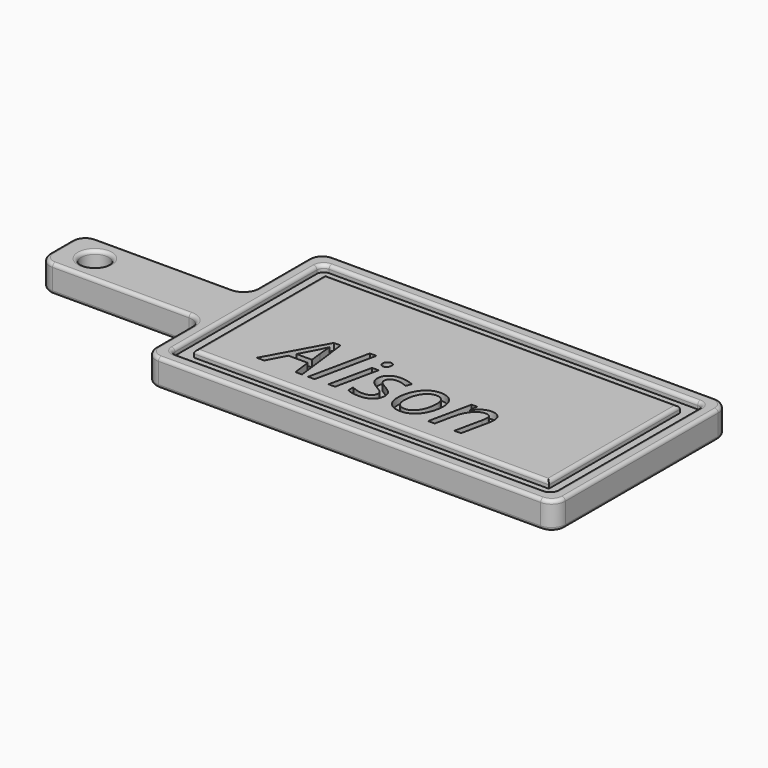
from build123d import *

# Parameters (mm, degrees)
F0_W         = 152.4
F0_H         = 50.8
F1_DEPTH     = 25.4
F2_R         = 12.7
F3_DEPTH     = 25.4
F5_DEPTH     = 6.35
F6_R         = 6.35
F7_R         = 12.7
F8_R         = 3.175
F9_TEXT_SIZE = 74.5518417615
F10_DEPTH    = 6.35


# Not quite as in the source:
# - Text() gives the source's letters only with a copy of the font that has no kerning and outlines rounded to 1/6400 em; it was checked with that copy


with BuildPart() as f1:
    # F0 (on Top) → F1 (new body)
    with BuildSketch(Plane.XY):
        Polygon((0, 67.31), (0, 0), (381, 0), (381, 203.2), (0, 203.2), (0, 118.11), align=None)
        with Locations((-76.2, 92.71)):
            Rectangle(F0_W, F0_H)
    extrude(amount=F1_DEPTH)

    # F2 (on face) → F3 (cut)
    with BuildSketch(Plane.XY.offset(25.4)):
        with Locations((-120.65, 92.71)):
            Circle(F2_R)
    extrude(amount=-F3_DEPTH, mode=Mode.SUBTRACT)

    # F4 (on face) → F5 (cut)
    with BuildSketch(Plane.XY.offset(25.4)):
        Polygon((12.6999939203, 67.31), (12.6999939203, 12.6999939203), (368.3000060797, 12.6999939203), (368.3000060797, 190.5000060797), (12.6999939203, 190.5000060797), (12.6999939203, 118.11), align=None)
        Polygon((25.4000002861, 67.31), (25.4000002861, 118.11), (25.4000002861, 177.7999997139), (355.5999997139, 177.7999997139), (355.5999997139, 25.4000002861), (25.4000002861, 25.4000002861), align=None, mode=Mode.SUBTRACT)
    extrude(amount=-F5_DEPTH, mode=Mode.SUBTRACT)

    # F6
    f6_edges = [f1.edges().sort_by_distance(p)[0] for p in [
        (12.699994, 190.500006, 22.225),
        (368.300006, 190.500006, 22.225),
        (368.300006, 12.699994, 22.225),
        (12.699994, 12.699994, 22.225),
    ]]
    fillet(f6_edges, radius=F6_R)

    # F7
    f7_edges = [f1.edges().sort_by_distance(p)[0] for p in [
        (381, 203.2, 12.7),
        (0, 203.2, 12.7),
        (381, 0, 12.7),
        (0, 0, 12.7),
        (-152.4, 67.31, 12.7),
        (-152.4, 118.11, 12.7),
        (0, 118.11, 12.7),
        (0, 67.31, 12.7),
    ]]
    fillet(f7_edges, radius=F7_R)

    # F8
    f8_edges = [f1.edges().sort_by_distance(p)[0] for p in [
        (190.5, 177.8, 25.4),
        (355.6, 101.6, 25.4),
        (190.5, 25.4, 25.4),
        (25.4, 101.6, 25.4),
        (0, 33.655, 25.4),
        (-3.719744, 63.590256, 25.4),
        (3.719744, 3.719744, 25.4),
        (-76.2, 67.31, 25.4),
        (190.5, 0, 25.4),
        (-148.680256, 71.029744, 25.4),
        (377.280256, 3.719744, 25.4),
        (-152.4, 92.71, 25.4),
        (381, 101.6, 25.4),
        (-148.680256, 114.390256, 25.4),
        (377.280256, 199.480256, 25.4),
        (-76.2, 118.11, 25.4),
        (190.5, 203.2, 25.4),
        (-3.719744, 121.829744, 25.4),
        (3.719744, 199.480256, 25.4),
        (0, 160.655, 25.4),
        (190.5, 12.699994, 25.4),
        (14.559866, 14.559866, 25.4),
        (366.440134, 14.559866, 25.4),
        (12.699994, 101.6, 25.4),
        (368.300006, 101.6, 25.4),
        (14.559866, 188.640134, 25.4),
        (366.440134, 188.640134, 25.4),
        (190.5, 190.500006, 25.4),
        (-133.35, 92.71, 25.4),
        (0, 33.655, 0),
        (-3.719744, 63.590256, 0),
        (3.719744, 3.719744, 0),
        (-76.2, 67.31, 0),
        (190.5, 0, 0),
        (-148.680256, 71.029744, 0),
        (377.280256, 3.719744, 0),
        (-152.4, 92.71, 0),
        (381, 101.6, 0),
        (-148.680256, 114.390256, 0),
        (377.280256, 199.480256, 0),
        (-76.2, 118.11, 0),
        (190.5, 203.2, 0),
        (-3.719744, 121.829744, 0),
        (3.719744, 199.480256, 0),
        (0, 160.655, 0),
        (-133.35, 92.71, 0),
    ]]
    fillet(f8_edges, radius=F8_R)

    # F9 (on face) → F10 (cut)
    with BuildSketch(Plane.XY.offset(25.4)):
        with Locations((73.0249939203, 44.2296545953)):
            Text('Alison', F9_TEXT_SIZE, font='Open Sans', font_style=FontStyle.ITALIC, text_align=(TextAlign.LEFT, TextAlign.BOTTOM))
    extrude(amount=-F10_DEPTH, mode=Mode.SUBTRACT)


solid = f1.part
